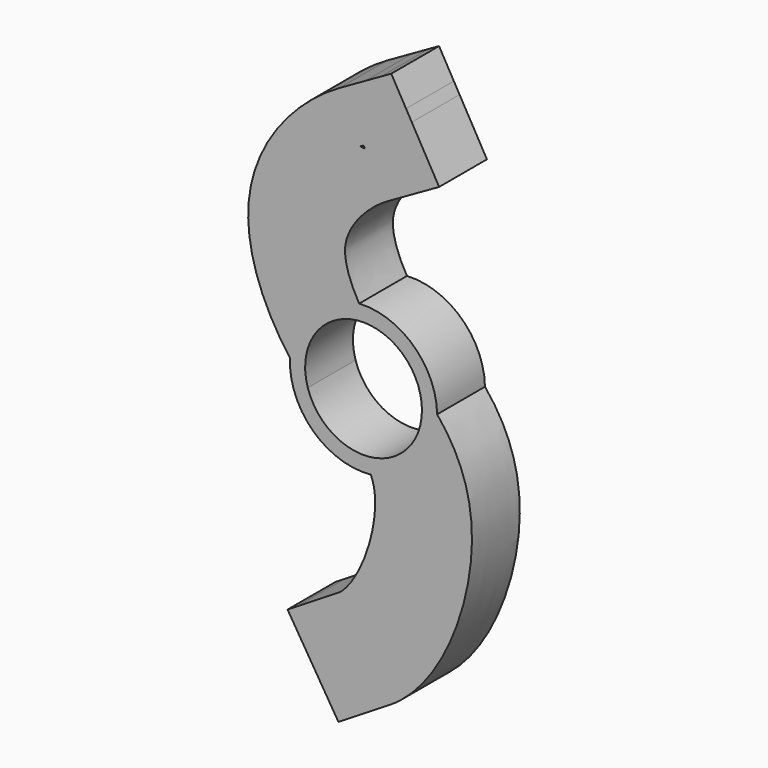
from build123d import *

# Parameters (mm, degrees)
F1_DEPTH = 12.7


# Not quite as in the source:
# - the dataset's text gives a spline's control points without its knots; the knots are read off the source's solid


with BuildPart() as f1:
    # F0 (on Front) → F1 (new body)
    with BuildSketch(Plane.XZ):
        with BuildLine():
            ThreePointArc((-11.8491375073, -3.6874569895), (-12.0319508259, 3.038347913), (-8.6778355467, 8.8709959385))
            add(Edge.make_bspline(
                [(-8.6778355467, 8.8709959385), (-9.2853744088, 9.7814260815), (-9.8597528454, 10.7272806041), (-10.3912226552, 11.6988451747)],
                knots=[0.2252802502, 0.2252802502, 0.2252802502, 0.2252802502, 0.2789767598, 0.2789767598, 0.2789767598, 0.2789767598], degree=3))
            ThreePointArc((-10.3912226552, 11.6988451747), (-14.1275753459, 6.7269682278), (-15.6320541614, 0.6923650678))
            add(Edge.make_bspline(
                [(-11.8491375073, -3.6874569895), (-12.0986304351, -3.4342357303), (-13.4209716173, -2.0574119677), (-14.6688396939, -0.5758176521), (-15.6320541614, 0.6923650678)],
                knots=[0.1107256969, 0.1107256969, 0.1107256969, 0.1107256969, 0.125, 0.187209023, 0.187209023, 0.187209023, 0.187209023], degree=3))
        make_face()
        with BuildLine():
            add(Edge.make_bspline(
                [(-8.6778355467, 8.8709959385), (-9.2853744088, 9.7814260815), (-9.8597528454, 10.7272806041), (-10.3912226552, 11.6988451747)],
                knots=[0.2252802502, 0.2252802502, 0.2252802502, 0.2252802502, 0.2789767598, 0.2789767598, 0.2789767598, 0.2789767598], degree=3))
            ThreePointArc((-8.6778355467, 8.8709959385), (-4.0348074378, 11.7354048782), (1.3880039263, 12.331781859))
            add(Edge.make_bspline(
                [(1.3880039263, 12.331781859), (1.1715122405, 12.5949393869), (0.3992065245, 13.5716380523), (-0.3737885205, 14.7019009055), (-0.8950079656, 15.5620901399), (-0.929649614, 15.6197387394)],
                knots=[0.1633568702, 0.1633568702, 0.1633568702, 0.1633568702, 0.1875, 0.25, 0.2544794081, 0.2544794081, 0.2544794081, 0.2544794081], degree=3))
            ThreePointArc((-0.929649614, 15.6197387394), (-5.9903162538, 14.4553311228), (-10.3912226552, 11.6988451747))
        make_face()
        with BuildLine():
            ThreePointArc((12.4096494196, 0), (11.5655450275, -4.4986183361), (9.1480638179, -8.3852446058))
            add(Edge.make_bspline(
                [(9.1480638179, -8.3852446058), (9.7633588854, -9.3122728001), (10.3114373795, -10.2956591108), (10.7802117804, -11.3414073492)],
                knots=[0.2554886882, 0.2554886882, 0.2554886882, 0.2554886882, 0.3234426707, 0.3234426707, 0.3234426707, 0.3234426707], degree=3))
            ThreePointArc((10.7802117804, -11.3414073492), (14.3791959444, -6.1708354931), (15.6473795471, 0))
            ThreePointArc((15.6473795471, 0), (15.6467175307, 0.1439347261), (15.6447315375, 0.2878572728))
            add(Edge.make_bspline(
                [(11.6109564261, 4.3800787194), (11.6883935226, 4.3126793989), (12.801065895, 3.3367304215), (14.1660004984, 2.000745319), (15.3850396401, 0.5978206791), (15.6447315375, 0.2878572728)],
                knots=[0.1203328038, 0.1203328038, 0.1203328038, 0.1203328038, 0.125, 0.1875, 0.2047375018, 0.2047375018, 0.2047375018, 0.2047375018], degree=3))
            ThreePointArc((11.6109564261, 4.3800787194), (12.208343405, 2.2261513923), (12.4096494196, 0))
        make_face()
        with BuildLine():
            add(Edge.make_bspline(
                [(9.1480638179, -8.3852446058), (9.7633588854, -9.3122728001), (10.3114373795, -10.2956591108), (10.7802117804, -11.3414073492)],
                knots=[0.2554886882, 0.2554886882, 0.2554886882, 0.2554886882, 0.3234426707, 0.3234426707, 0.3234426707, 0.3234426707], degree=3))
            ThreePointArc((9.1480638179, -8.3852446058), (4.7241366094, -11.4752748121), (-0.5930675386, -12.3954697213))
            add(Edge.make_bspline(
                [(-0.5930675386, -12.3954697213), (-0.5422251349, -12.4502827191), (-0.0893674975, -12.9460413617), (0.6470698049, -13.8821382909), (1.2271907242, -14.8823314511), (1.4942386676, -15.4627127324), (1.5418348503, -15.5712309078)],
                knots=[0.1797309234, 0.1797309234, 0.1797309234, 0.1797309234, 0.1875, 0.25, 0.3125, 0.326664828, 0.326664828, 0.326664828, 0.326664828], degree=3))
            ThreePointArc((1.5418348503, -15.5712309078), (6.5139128123, -14.2270666887), (10.7802117804, -11.3414073492))
        make_face()
        with BuildLine():
            ThreePointArc((-15.6320541614, 0.6923650678), (-14.1275753459, 6.7269682278), (-10.3912226552, 11.6988451747))
            add(Edge.make_bspline(
                [(-10.3912226552, 11.6988451747), (-12.8029404637, 16.1076366694), (-17.2123471815, 30.3566232389), (-6.6813074108, 41.4558396662), (-0.6964705023, 45.0986841551)],
                knots=[0.2789767598, 0.2789767598, 0.2789767598, 0.2789767598, 0.5226422061, 0.9820627069, 0.9820627069, 0.9820627069, 0.9820627069], degree=3))
            add(Edge.make_bspline(
                [(-0.6964705023, 45.0986841551), (-0.4628027101, 45.240912831), (-0.2305015334, 45.377638856), (0, 45.5087274313)],
                knots=[0.9820627069, 0.9820627069, 0.9820627069, 0.9820627069, 1, 1, 1, 1], degree=3))
            Line((0, 45.5087274313), (-5.1482294751, 54.5611928011))
            add(Edge.make_bspline(
                [(-15.6320541614, 0.6923650678), (-15.636559509, 0.6982968766), (-16.6085403024, 1.978641132), (-18.442751654, 4.6616170097), (-20.8194846225, 9.0288333995), (-22.7427732281, 13.7302890055), (-23.866202795, 17.9262301222), (-24.3194859098, 21.0117640249), (-24.4669610536, 22.8159468829), (-24.5172239147, 24.1889005784), (-24.502571598, 25.579766526), (-24.388031674, 27.4585942739), (-24.0729268068, 29.7376311161), (-23.4541878049, 32.3541134778), (-22.6288454178, 34.8352906061), (-21.6295067826, 37.1769157355), (-20.1035209307, 40.1126812586), (-17.8979428955, 43.4406369139), (-14.9345931184, 46.9263269169), (-11.7707761701, 49.9398108312), (-8.4930608318, 52.5043610495), (-6.269432358, 53.9235532749), (-5.1482294751, 54.5611928011)],
                knots=[0.187209023, 0.187209023, 0.187209023, 0.187209023, 0.1875, 0.25, 0.3125, 0.375, 0.4375, 0.46875, 0.484375, 0.5, 0.515625, 0.53125, 0.5625, 0.59375, 0.625, 0.65625, 0.6875, 0.75, 0.8125, 0.875, 0.9375, 1, 1, 1, 1], degree=3))
        make_face()
        with BuildLine():
            add(Edge.make_bspline(
                [(-10.3912226552, 11.6988451747), (-12.8029404637, 16.1076366694), (-17.2123471815, 30.3566232389), (-6.6813074108, 41.4558396662), (-0.6964705023, 45.0986841551)],
                knots=[0.2789767598, 0.2789767598, 0.2789767598, 0.2789767598, 0.5226422061, 0.9820627069, 0.9820627069, 0.9820627069, 0.9820627069], degree=3))
            ThreePointArc((-10.3912226552, 11.6988451747), (-5.9903162538, 14.4553311228), (-0.929649614, 15.6197387394))
            add(Edge.make_bspline(
                [(-0.929649614, 15.6197387394), (-1.378353745, 16.3664458385), (-2.2350758783, 17.9598118494), (-3.2119329355, 20.3694931918), (-3.7060132508, 22.267017983), (-3.8731893948, 23.4296691454), (-3.9222634293, 24.0367170821), (-3.9374083126, 24.4611674633), (-3.9326943692, 24.8538568084), (-3.9034333763, 25.3305962326), (-3.8198337247, 25.9465502567), (-3.6393425731, 26.7167285079), (-3.3722246374, 27.525901957), (-3.0139222068, 28.3697964463), (-2.4132338328, 29.5303307169), (-1.436511786, 31.0185840281), (0.0361873799, 32.7590338295), (1.7057339174, 34.3516547718), (3.4394466992, 35.7061480035), (4.5298073789, 36.3967620304), (5.0226628601, 36.6770539743)],
                knots=[0.2544794081, 0.2544794081, 0.2544794081, 0.2544794081, 0.3125, 0.375, 0.4375, 0.46875, 0.484375, 0.5, 0.515625, 0.53125, 0.5625, 0.59375, 0.625, 0.65625, 0.6875, 0.75, 0.8125, 0.875, 0.9375, 1, 1, 1, 1], degree=3))
            Line((5.0226628601, 36.6770539743), (0.3061173234, 44.9704615124))
            Line((0.3061173234, 44.9704615124), (-0.6964705023, 45.0986841551))
        make_face()
        with BuildLine():
            add(Edge.make_bspline(
                [(1.3880039263, 12.331781859), (1.1715122405, 12.5949393869), (0.3992065245, 13.5716380523), (-0.3737885205, 14.7019009055), (-0.8950079656, 15.5620901399), (-0.929649614, 15.6197387394)],
                knots=[0.1633568702, 0.1633568702, 0.1633568702, 0.1633568702, 0.1875, 0.25, 0.2544794081, 0.2544794081, 0.2544794081, 0.2544794081], degree=3))
            ThreePointArc((1.3880039263, 12.331781859), (7.6190969455, 9.7953438148), (11.6109564261, 4.3800787194))
            add(Edge.make_bspline(
                [(11.6109564261, 4.3800787194), (11.6883935226, 4.3126793989), (12.801065895, 3.3367304215), (14.1660004984, 2.000745319), (15.3850396401, 0.5978206791), (15.6447315375, 0.2878572728)],
                knots=[0.1203328038, 0.1203328038, 0.1203328038, 0.1203328038, 0.125, 0.1875, 0.2047375018, 0.2047375018, 0.2047375018, 0.2047375018], degree=3))
            ThreePointArc((15.6447315375, 0.2878572728), (10.625443818, 11.4865325647), (-0.929649614, 15.6197387394))
        make_face()
        with BuildLine():
            ThreePointArc((-0.5930675386, -12.3954697213), (-7.5933844915, -9.8152896381), (-11.8491375073, -3.6874569895))
            add(Edge.make_bspline(
                [(-11.8491375073, -3.6874569895), (-12.0986304351, -3.4342357303), (-13.4209716173, -2.0574119677), (-14.6688396939, -0.5758176521), (-15.6320541614, 0.6923650678)],
                knots=[0.1107256969, 0.1107256969, 0.1107256969, 0.1107256969, 0.125, 0.187209023, 0.187209023, 0.187209023, 0.187209023], degree=3))
            ThreePointArc((-15.6320541614, 0.6923650678), (-10.7591685819, -11.3613721934), (1.5418348503, -15.5712309078))
            add(Edge.make_bspline(
                [(-0.5930675386, -12.3954697213), (-0.5422251349, -12.4502827191), (-0.0893674975, -12.9460413617), (0.6470698049, -13.8821382909), (1.2271907242, -14.8823314511), (1.4942386676, -15.4627127324), (1.5418348503, -15.5712309078)],
                knots=[0.1797309234, 0.1797309234, 0.1797309234, 0.1797309234, 0.1875, 0.25, 0.3125, 0.326664828, 0.326664828, 0.326664828, 0.326664828], degree=3))
        make_face()
        with BuildLine():
            ThreePointArc((15.6473795471, 0), (14.3791959444, -6.1708354931), (10.7802117804, -11.3414073492))
            add(Edge.make_bspline(
                [(10.7802117804, -11.3414073492), (11.6264835061, -13.229281697), (14.8682711517, -24.7617360554), (8.08607989, -43.5501283525), (0, -48.5415357893)],
                knots=[0.3234426707, 0.3234426707, 0.3234426707, 0.3234426707, 0.446119024, 1, 1, 1, 1], degree=3))
            Line((0, -48.5415357893), (5.4701533549, -57.4031840516))
            add(Edge.make_bspline(
                [(15.6447315375, 0.2878572728), (16.3266345282, -0.5260494212), (17.8871346304, -2.5735124946), (19.6343071308, -5.5649885279), (20.9151883898, -8.5103892259), (21.7132531018, -10.8356150551), (22.3344664493, -13.2646623418), (22.6966343535, -15.3618244109), (22.8903478004, -17.0806012193), (23.0186382679, -18.796096541), (23.0662198627, -20.9378919201), (22.9630569039, -23.5038601417), (22.6309798906, -26.9181954555), (21.878352145, -31.1655622837), (20.48723974, -36.1834140821), (18.6296401775, -41.0581085457), (16.2998809407, -45.718972551), (13.452397619, -50.0911504281), (10.5555341156, -53.4229665407), (7.8168542439, -55.8195818603), (6.2831768326, -56.9013176976), (5.4701533549, -57.4031840516)],
                knots=[0.2047375018, 0.2047375018, 0.2047375018, 0.2047375018, 0.25, 0.3125, 0.34375, 0.375, 0.40625, 0.4375, 0.453125, 0.46875, 0.5, 0.53125, 0.5625, 0.625, 0.6875, 0.75, 0.8125, 0.875, 0.9375, 0.96875, 1, 1, 1, 1], degree=3))
            ThreePointArc((15.6447315375, 0.2878572728), (15.6467175307, 0.1439347261), (15.6473795471, 0))
        make_face()
        with BuildLine():
            add(Edge.make_bspline(
                [(10.7802117804, -11.3414073492), (11.6264835061, -13.229281697), (14.8682711517, -24.7617360554), (8.08607989, -43.5501283525), (0, -48.5415357893)],
                knots=[0.3234426707, 0.3234426707, 0.3234426707, 0.3234426707, 0.446119024, 1, 1, 1, 1], degree=3))
            ThreePointArc((10.7802117804, -11.3414073492), (6.5139128123, -14.2270666887), (1.5418348503, -15.5712309078))
            add(Edge.make_bspline(
                [(1.5418348503, -15.5712309078), (1.5992438757, -15.7021221335), (1.7544783645, -16.0777122744), (1.9777658515, -16.7272947355), (2.1915014853, -17.5590215657), (2.3250200741, -18.3262912642), (2.4004010179, -18.9913445586), (2.4554405815, -19.718914297), (2.4799779419, -20.7306801507), (2.4275831434, -22.0764789614), (2.2418770735, -24.0043519572), (1.7882246185, -26.5906690812), (0.9098712215, -29.7617893454), (-0.2521338933, -32.8032773219), (-1.6209855373, -35.5242995778), (-3.0809606838, -37.7381050829), (-4.2238837122, -39.0131375196), (-4.9541458564, -39.6412317653), (-5.2286217969, -39.8292882956), (-5.3367351858, -39.8960249567)],
                knots=[0.326664828, 0.326664828, 0.326664828, 0.326664828, 0.34375, 0.375, 0.40625, 0.4375, 0.453125, 0.46875, 0.5, 0.53125, 0.5625, 0.625, 0.6875, 0.75, 0.8125, 0.875, 0.9375, 0.96875, 1, 1, 1, 1], degree=3))
            Line((-5.3367351858, -39.8960249567), (0, -48.5415357893))
        make_face()
        Polygon((-13.237771211, -46.922370502), (0, -48.5415357893), (-5.3367351858, -39.8960249567), (-14.1983836254, -45.366178421), align=None)
        Polygon((5.4701533549, -57.4031840516), (0, -48.5415357893), (-13.237771211, -46.922370502), (-7.8223193044, -55.6954024197), align=None)
        Polygon((-5.1482294751, 54.5611928011), (0, 45.5087274313), (0.3061173234, 44.9704615124), (12.9110272843, 43.3583983844), (7.1709556817, 53.4515381045), align=None)
        Polygon((12.9110272843, 43.3583983844), (0.3061173234, 44.9704615124), (5.0226628601, 36.6770539743), (13.8543363917, 41.6997168768), align=None)
        Polygon((0.3715664821, 57.7003571152), (-5.1482294751, 54.5611928011), (7.1709556817, 53.4515381045), (3.6834440565, 59.5838557036), align=None)
        Polygon((0.0667090845, -60.7386435427), (5.4701533549, -57.4031840516), (-7.8223193044, -55.6954024197), (-3.3914950846, -62.8733375159), align=None)
        Polygon((-7.8223193044, -55.6954024197), (-13.237771211, -46.922370502), (-16.1436237266, -46.566943939), (-10.7401794562, -55.3205234864), align=None)
        Polygon((-16.1436237266, -46.566943939), (-13.237771211, -46.922370502), (-14.1983836254, -45.366178421), align=None)
        Polygon((7.1709556817, 53.4515381045), (12.9110272843, 43.3583983844), (16.0622547746, 42.9553826024), (10.2507519709, 53.1741244303), align=None)
        Polygon((16.0622547746, 42.9553826024), (12.9110272843, 43.3583983844), (13.8543363917, 41.6997168768), align=None)
        Polygon((3.6834440565, 59.5838557036), (7.1709556817, 53.4515381045), (10.2507519709, 53.1741244303), (9.0305267534, 55.319725472), (5.8913624394, 60.8395214293), align=None)
        Polygon((-3.3914950846, -62.8733375159), (-7.8223193044, -55.6954024197), (-10.7401794562, -55.3205234864), (-8.672194677, -58.6706587635), (-5.3367351858, -64.0741030339), align=None)
    extrude(amount=F1_DEPTH)


solid = f1.part
